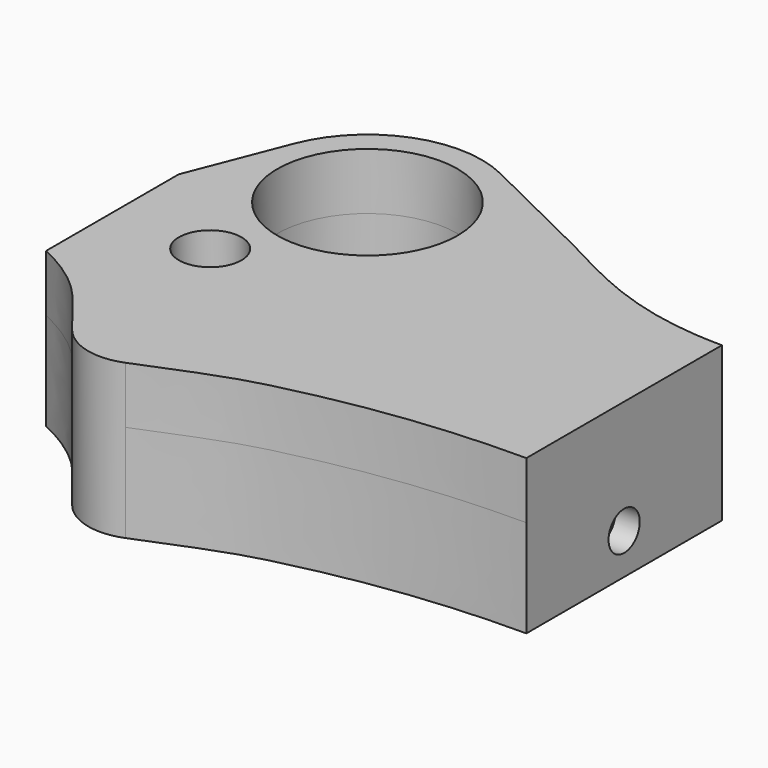
from build123d import *

# Parameters (mm, degrees)
F0_R           = 4.15
F1_DEPTH       = 12
F2_DEPTH       = 3.16
F3_DEPTH       = 7
F6_D           = 4.8
F6_DEPTH       = 15
F6_CBORE_D     = 7.7
F6_CBORE_DEPTH = 7
F6_TIP         = 1.4420654857
F7_D           = 4.8
F7_DEPTH       = 10
F7_TIP         = 1.4420654857
F8_DEPTH       = 2


# Not quite as in the source:
# - after a boolean that leaves OpenCascade's solid faulty, fix() repairs it


with BuildPart() as f1:
    # F0 (on Top) → F1 (new body)
    with BuildSketch(Plane.XY):
        with BuildLine():
            Line((30, 10.2), (30, -10.2))
            Line((30, -10.2), (-30, -10.2))
            add(Edge.make_bspline(
                [(-17.7992275989, -21.4464761661), (-20.8859294653, -17.5595451146), (-21.6980138001, -16.2221621605), (-25.6317793117, -12.2553748449), (-30, -10.2)],
                knots=[0, 0, 0, 0, 0.4674468376, 1, 1, 1, 1], degree=3))
            ThreePointArc((-17.7992275989, -21.4464761661), (-14.003054565, -23.9189229101), (-9.4830172376, -23.6136604591))
            add(Edge.make_bspline(
                [(-9.4830172376, -23.6136604591), (0, -19.7179064316), (4.4370511503, -18.4021307002), (20.4163611322, -15.0439910263), (33, -15.0439910263)],
                knots=[0, 0, 0, 0, 0.4385632438, 1, 1, 1, 1], degree=3))
            Line((33, -15.0439910263), (33, 15.0439910263))
            add(Edge.make_bspline(
                [(-5.9802875731, 29.6540577416), (4.8586864574, 24.3264938357), (9.2455528778, 22.3735984932), (22.4546817712, 15.0439910263), (33, 15.0439910263)],
                knots=[0.0105896754, 0.0105896754, 0.0105896754, 0.0105896754, 0.4824749826, 1, 1, 1, 1], degree=3))
            ThreePointArc((-5.9802875731, 29.6540577416), (-0.2311248394, 24.4535915766), (1.9, 17))
            ThreePointArc((1.9, 17), (1.4559897714, 13.4894525551), (0.1519229272, 10.2))
            Line((0.1519229272, 10.2), (30, 10.2))
        make_face()
        with Locations((-12.2, -17)):
            Circle(F0_R, mode=Mode.SUBTRACT)
        with BuildLine():
            Line((-3.4267451878, 10.2), (0.1519229272, 10.2))
            ThreePointArc((0.1519229272, 10.2), (1.4559897714, 13.4894525551), (1.9, 17))
            ThreePointArc((1.9, 17), (-0.2311248394, 24.4535915766), (-5.9802875731, 29.6540577416))
            ThreePointArc((-5.9802875731, 29.6540577416), (-17.3060634553, 30.1429873313), (-25.3312422306, 22.1361928977))
            ThreePointArc((-25.3312422306, 22.1361928977), (-26.2700427092, 16.0813607005), (-24.5519229272, 10.2))
            Line((-24.5519229272, 10.2), (-20.9732548122, 10.2))
            ThreePointArc((-20.9732548122, 10.2), (-15.7935269294, 27.5022171092), (-1.1, 17))
            ThreePointArc((-1.1, 17), (-1.6977828908, 13.4064730706), (-3.4267451878, 10.2))
        make_face()
        with BuildLine():
            Line((-25.3312422306, 22.1361928977), (-30, 10.2))
            Line((-30, 10.2), (-24.5519229272, 10.2))
            ThreePointArc((-24.5519229272, 10.2), (-26.2700427092, 16.0813607005), (-25.3312422306, 22.1361928977))
        make_face()
    extrude(amount=-F1_DEPTH)

    # F0 (on Top) → F2 (join)
    with BuildSketch(Plane.XY):
        with BuildLine():
            Line((-30, -10.2), (30, -10.2))
            Line((30, -10.2), (30, 10.2))
            Line((30, 10.2), (0.1519229272, 10.2))
            ThreePointArc((0.1519229272, 10.2), (-12.2, 2.9), (-24.5519229272, 10.2))
            Line((-24.5519229272, 10.2), (-30, 10.2))
            Line((-30, 10.2), (-30, -10.2))
        make_face()
        with BuildLine():
            ThreePointArc((-24.5519229272, 10.2), (-12.2, 2.9), (0.1519229272, 10.2))
            Line((0.1519229272, 10.2), (-3.4267451878, 10.2))
            ThreePointArc((-3.4267451878, 10.2), (-12.2, 5.9), (-20.9732548122, 10.2))
            Line((-20.9732548122, 10.2), (-24.5519229272, 10.2))
        make_face()
        with BuildLine():
            ThreePointArc((-20.9732548122, 10.2), (-12.2, 5.9), (-3.4267451878, 10.2))
            Line((-3.4267451878, 10.2), (-20.9732548122, 10.2))
        make_face()
        with Locations((-12.2, -17)):
            Circle(F0_R)
    extrude(amount=-F2_DEPTH)

    # F0 (on Top) → F3 (join)
    with BuildSketch(Plane.XY):
        with BuildLine():
            Line((-3.4267451878, 10.2), (0.1519229272, 10.2))
            ThreePointArc((0.1519229272, 10.2), (1.4559897714, 13.4894525551), (1.9, 17))
            ThreePointArc((1.9, 17), (-0.2311248394, 24.4535915766), (-5.9802875731, 29.6540577416))
            ThreePointArc((-5.9802875731, 29.6540577416), (-17.3060634553, 30.1429873313), (-25.3312422306, 22.1361928977))
            ThreePointArc((-25.3312422306, 22.1361928977), (-26.2700427092, 16.0813607005), (-24.5519229272, 10.2))
            Line((-24.5519229272, 10.2), (-20.9732548122, 10.2))
            ThreePointArc((-20.9732548122, 10.2), (-15.7935269294, 27.5022171092), (-1.1, 17))
            ThreePointArc((-1.1, 17), (-1.6977828908, 13.4064730706), (-3.4267451878, 10.2))
        make_face()
        with BuildLine():
            ThreePointArc((-24.5519229272, 10.2), (-12.2, 2.9), (0.1519229272, 10.2))
            Line((0.1519229272, 10.2), (-3.4267451878, 10.2))
            ThreePointArc((-3.4267451878, 10.2), (-12.2, 5.9), (-20.9732548122, 10.2))
            Line((-20.9732548122, 10.2), (-24.5519229272, 10.2))
        make_face()
        with BuildLine():
            Line((30, 10.2), (30, -10.2))
            Line((30, -10.2), (-30, -10.2))
            add(Edge.make_bspline(
                [(-17.7992275989, -21.4464761661), (-20.8859294653, -17.5595451146), (-21.6980138001, -16.2221621605), (-25.6317793117, -12.2553748449), (-30, -10.2)],
                knots=[0, 0, 0, 0, 0.4674468376, 1, 1, 1, 1], degree=3))
            ThreePointArc((-17.7992275989, -21.4464761661), (-14.003054565, -23.9189229101), (-9.4830172376, -23.6136604591))
            add(Edge.make_bspline(
                [(-9.4830172376, -23.6136604591), (0, -19.7179064316), (4.4370511503, -18.4021307002), (20.4163611322, -15.0439910263), (33, -15.0439910263)],
                knots=[0, 0, 0, 0, 0.4385632438, 1, 1, 1, 1], degree=3))
            Line((33, -15.0439910263), (33, 15.0439910263))
            add(Edge.make_bspline(
                [(-5.9802875731, 29.6540577416), (4.8586864574, 24.3264938357), (9.2455528778, 22.3735984932), (22.4546817712, 15.0439910263), (33, 15.0439910263)],
                knots=[0.0105896754, 0.0105896754, 0.0105896754, 0.0105896754, 0.4824749826, 1, 1, 1, 1], degree=3))
            ThreePointArc((-5.9802875731, 29.6540577416), (-0.2311248394, 24.4535915766), (1.9, 17))
            ThreePointArc((1.9, 17), (1.4559897714, 13.4894525551), (0.1519229272, 10.2))
            Line((0.1519229272, 10.2), (30, 10.2))
        make_face()
        with Locations((-12.2, -17)):
            Circle(F0_R, mode=Mode.SUBTRACT)
        with BuildLine():
            Line((-30, -10.2), (30, -10.2))
            Line((30, -10.2), (30, 10.2))
            Line((30, 10.2), (0.1519229272, 10.2))
            ThreePointArc((0.1519229272, 10.2), (-12.2, 2.9), (-24.5519229272, 10.2))
            Line((-24.5519229272, 10.2), (-30, 10.2))
            Line((-30, 10.2), (-30, -10.2))
        make_face()
        with BuildLine():
            Line((-25.3312422306, 22.1361928977), (-30, 10.2))
            Line((-30, 10.2), (-24.5519229272, 10.2))
            ThreePointArc((-24.5519229272, 10.2), (-26.2700427092, 16.0813607005), (-25.3312422306, 22.1361928977))
        make_face()
        with Locations((-12.2, -17)):
            Circle(F0_R)
    extrude(amount=F3_DEPTH)

    # F6
    with Locations(Plane.XY.offset(7)):
        with Locations((-17.9568603635, 0)):
            CounterBoreHole(F6_D / 2, F6_CBORE_D / 2, F6_CBORE_DEPTH, depth=F6_DEPTH)
            with Locations((0, 0, -(F6_DEPTH + F6_TIP / 2))):  # 118° drill point
                Cone(0, F6_D / 2, F6_TIP, mode=Mode.SUBTRACT)

    # F7
    with Locations(Plane.YZ.offset(33)):
        with Locations((0, -7)):
            Hole(F7_D / 2, depth=F7_DEPTH)
            with Locations((0, 0, -(F7_DEPTH + F7_TIP / 2))):  # 118° drill point
                Cone(0, F7_D / 2, F7_TIP, mode=Mode.SUBTRACT)

    add(f1.part.fix(), mode=Mode.REPLACE)

    # F8 (cut): a face of the model
    f8_faces = [f1.faces().sort_by_distance(p)[0] for p in [
        (-12.2, -17, -3.16),
    ]]
    extrude(f8_faces, amount=-F8_DEPTH, mode=Mode.SUBTRACT)


solid = f1.part
